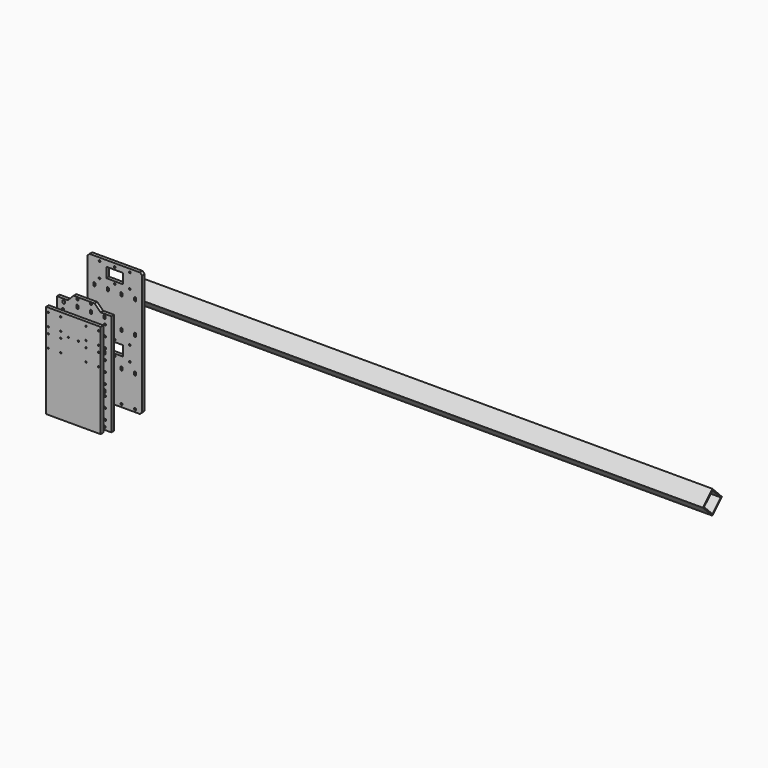
from build123d import *

# Parameters (mm, degrees)
F2_DEPTH  = 1380
F3_T      = -2.5
F4_R      = 2.25
F4_R_2    = 2.5
F4_R_3    = 2.5703929726
F4_R_4    = 2.4889347238
F5_DEPTH  = 8
F7_R      = 2.5
F7_R_2    = 2.05
F7_W      = 40
F7_H      = 24
F8_DEPTH  = 8
F10_W     = 130
F10_H     = 225
F10_R     = 1.65
F11_DEPTH = 8


# Not quite as in the source:
# - a feature names something its author has since deleted; it is built from what else it names


with BuildPart() as f2:
    # F1 (on Right) → F2 (new body)
    with BuildSketch(Plane.YZ):
        Polygon((165.6129737569, 100.5009111076), (137.3287025094, 128.785182355), (109.0444312619, 100.5009111076), (137.3287025094, 72.2166398601), align=None)
    extrude(amount=F2_DEPTH)

    # F3
    f3_openings = [f2.faces().sort_by_distance(p)[0] for p in [
        (0, 137.328703, 100.500911),
        (1380, 137.328703, 100.500911),
    ]]
    offset(amount=F3_T, openings=f3_openings)


with BuildPart() as f5:
    # F4 (on Front) → F5 (new body)
    with BuildSketch(Plane.XZ):
        Polygon((65, -121.7), (65, 121.7), (39, 121.7), (25, 135.7), (-25, 135.7), (-39, 121.7), (-65, 121.7), (-65, -121.7), (-45, -121.7), (-34, -131.8), (34, -131.8), (45, -121.7), align=None)
        with Locations((-50, -100.09)):
            Circle(F4_R, mode=Mode.SUBTRACT)
        with Locations((-48.5, -115.09)):
            Circle(F4_R_2, mode=Mode.SUBTRACT)
        with Locations((-50, -75.09)):
            Circle(F4_R, mode=Mode.SUBTRACT)
        with Locations((-16.18, -127.59)):
            Circle(F4_R_2, mode=Mode.SUBTRACT)
        with Locations((-16.18, -115.09)):
            Circle(F4_R_2, mode=Mode.SUBTRACT)
        with Locations((-50, -50.09)):
            Circle(F4_R, mode=Mode.SUBTRACT)
        with BuildLine():
            Line((-46, -38.512), (-46, -42.512))
            ThreePointArc((-46, -42.512), (-48.5, -45.012), (-51, -42.512))
            Line((-51, -42.512), (-51, -38.512))
            ThreePointArc((-51, -38.512), (-48.5, -36.012), (-46, -38.512))
        make_face(mode=Mode.SUBTRACT)
        with Locations((-50, -25.09)):
            Circle(F4_R, mode=Mode.SUBTRACT)
        with Locations((-50, -0.09)):
            Circle(F4_R, mode=Mode.SUBTRACT)
        with BuildLine():
            Line((-13.68, -38.512), (-13.68, -42.512))
            ThreePointArc((-13.68, -42.512), (-16.18, -45.012), (-18.68, -42.512))
            Line((-18.68, -42.512), (-18.68, -38.512))
            ThreePointArc((-18.68, -38.512), (-16.18, -36.012), (-13.68, -38.512))
        make_face(mode=Mode.SUBTRACT)
        with Locations((16.18, -127.59)):
            Circle(F4_R_2, mode=Mode.SUBTRACT)
        with Locations((16.18, -115.09)):
            Circle(F4_R_2, mode=Mode.SUBTRACT)
        with Locations((48.5, -115.09)):
            Circle(F4_R_2, mode=Mode.SUBTRACT)
        with Locations((50, -100.09)):
            Circle(F4_R, mode=Mode.SUBTRACT)
        with Locations((50, -75.09)):
            Circle(F4_R, mode=Mode.SUBTRACT)
        with BuildLine():
            Line((18.68, -38.512), (18.68, -42.512))
            ThreePointArc((18.68, -42.512), (16.18, -45.012), (13.68, -42.512))
            Line((13.68, -42.512), (13.68, -38.512))
            ThreePointArc((13.68, -38.512), (16.18, -36.012), (18.68, -38.512))
        make_face(mode=Mode.SUBTRACT)
        with BuildLine():
            Line((51, -38.512), (51, -42.512))
            ThreePointArc((51, -42.512), (48.5, -45.012), (46, -42.512))
            Line((46, -42.512), (46, -38.512))
            ThreePointArc((46, -38.512), (48.5, -36.012), (51, -38.512))
        make_face(mode=Mode.SUBTRACT)
        with Locations((50, -50.09)):
            Circle(F4_R, mode=Mode.SUBTRACT)
        with Locations((50, -25.09)):
            Circle(F4_R, mode=Mode.SUBTRACT)
        with Locations((50, -0.09)):
            Circle(F4_R, mode=Mode.SUBTRACT)
        with Locations((-50, 24.91)):
            Circle(F4_R, mode=Mode.SUBTRACT)
        with Locations((-50, 49.91)):
            Circle(F4_R, mode=Mode.SUBTRACT)
        with BuildLine():
            Line((-51, 38.512), (-51, 42.512))
            ThreePointArc((-51, 42.512), (-48.5, 45.012), (-46, 42.512))
            Line((-46, 42.512), (-46, 38.512))
            ThreePointArc((-46, 38.512), (-48.5, 36.012), (-51, 38.512))
        make_face(mode=Mode.SUBTRACT)
        with BuildLine():
            Line((-18.68, 38.512), (-18.68, 42.512))
            ThreePointArc((-18.68, 42.512), (-16.18, 45.012), (-13.68, 42.512))
            Line((-13.68, 42.512), (-13.68, 38.512))
            ThreePointArc((-13.68, 38.512), (-16.18, 36.012), (-18.68, 38.512))
        make_face(mode=Mode.SUBTRACT)
        with Locations((-50, 74.91)):
            Circle(F4_R, mode=Mode.SUBTRACT)
        with Locations((-50, 99.91)):
            Circle(F4_R, mode=Mode.SUBTRACT)
        with BuildLine():
            Line((-51, 113.09), (-51, 117.09))
            ThreePointArc((-51, 117.09), (-48.5, 119.59), (-46, 117.09))
            Line((-46, 117.09), (-46, 113.09))
            ThreePointArc((-46, 113.09), (-48.5, 110.59), (-51, 113.09))
        make_face(mode=Mode.SUBTRACT)
        with BuildLine():
            Line((-18.68, 113.09), (-18.68, 117.09))
            ThreePointArc((-18.68, 117.09), (-16.18, 119.59), (-13.68, 117.09))
            Line((-13.68, 117.09), (-13.68, 113.09))
            ThreePointArc((-13.68, 113.09), (-16.18, 110.59), (-18.68, 113.09))
        make_face(mode=Mode.SUBTRACT)
        with Locations((-16.18, 130.7444572449)):
            Circle(F4_R_3, mode=Mode.SUBTRACT)
        with BuildLine():
            Line((13.68, 38.512), (13.68, 42.512))
            ThreePointArc((13.68, 42.512), (16.18, 45.012), (18.68, 42.512))
            Line((18.68, 42.512), (18.68, 38.512))
            ThreePointArc((18.68, 38.512), (16.18, 36.012), (13.68, 38.512))
        make_face(mode=Mode.SUBTRACT)
        with Locations((50, 24.91)):
            Circle(F4_R, mode=Mode.SUBTRACT)
        with BuildLine():
            Line((46, 38.512), (46, 42.512))
            ThreePointArc((46, 42.512), (48.5, 45.012), (51, 42.512))
            Line((51, 42.512), (51, 38.512))
            ThreePointArc((51, 38.512), (48.5, 36.012), (46, 38.512))
        make_face(mode=Mode.SUBTRACT)
        with Locations((50, 49.91)):
            Circle(F4_R, mode=Mode.SUBTRACT)
        with BuildLine():
            Line((13.68, 113.09), (13.68, 117.09))
            ThreePointArc((13.68, 117.09), (16.18, 119.59), (18.68, 117.09))
            Line((18.68, 117.09), (18.68, 113.09))
            ThreePointArc((18.68, 113.09), (16.18, 110.59), (13.68, 113.09))
        make_face(mode=Mode.SUBTRACT)
        with Locations((16.18, 132.09)):
            Circle(F4_R_4, mode=Mode.SUBTRACT)
        with Locations((50, 74.91)):
            Circle(F4_R, mode=Mode.SUBTRACT)
        with Locations((50, 99.91)):
            Circle(F4_R, mode=Mode.SUBTRACT)
        with BuildLine():
            Line((46, 113.09), (46, 117.09))
            ThreePointArc((46, 117.09), (48.5, 119.59), (51, 117.09))
            Line((51, 117.09), (51, 113.09))
            ThreePointArc((51, 113.09), (48.5, 110.59), (46, 113.09))
        make_face(mode=Mode.SUBTRACT)
    extrude(amount=F5_DEPTH)


with BuildPart() as f8:
    # F7 (on offset) → F8 (new body)
    with BuildSketch(Plane.XZ.offset(-83)):
        Polygon((60, 175.09), (-60, 175.09), (-65, 170.09), (-65, -116.7), (-60, -121.7), (60, -121.7), (65, -116.7), (65, 170.09), align=None)
        with Locations((-48.51, -115.2)):
            Circle(F7_R, mode=Mode.SUBTRACT)
        with Locations((-16.17, -115.2)):
            Circle(F7_R, mode=Mode.SUBTRACT)
        with BuildLine():
            Line((-46.01, -38.73), (-46.01, -42.73))
            ThreePointArc((-46.01, -42.73), (-48.51, -45.23), (-51.01, -42.73))
            Line((-51.01, -42.73), (-51.01, -38.9570118877))
            ThreePointArc((-51.01, -38.9570118877), (-48.6287763125, -36.2274246067), (-46.01, -38.73))
        make_face(mode=Mode.SUBTRACT)
        with Locations((-36, -20)):
            Circle(F7_R_2, mode=Mode.SUBTRACT)
        with Locations((-36, 15)):
            Circle(F7_R_2, mode=Mode.SUBTRACT)
        with BuildLine():
            Line((-13.67, -38.73), (-13.67, -42.73))
            ThreePointArc((-13.67, -42.73), (-16.17, -45.23), (-18.67, -42.73))
            Line((-18.67, -42.73), (-18.67, -39.0080270306))
            ThreePointArc((-18.67, -39.0080270306), (-16.3169581646, -36.2261380315), (-13.67, -38.73))
        make_face(mode=Mode.SUBTRACT)
        with Locations((16.17, -115.2)):
            Circle(F7_R, mode=Mode.SUBTRACT)
        with Locations((48.51, -115.2)):
            Circle(F7_R, mode=Mode.SUBTRACT)
        with BuildLine():
            Line((18.67, -38.73), (18.67, -42.73))
            ThreePointArc((18.67, -42.73), (16.17, -45.23), (13.67, -42.73))
            Line((13.67, -42.73), (13.67, -39.0075720796))
            ThreePointArc((13.67, -39.0075720796), (13.6584102142, -38.8690010606), (13.6545429641, -38.73))
            ThreePointArc((13.6545429641, -38.73), (16.1545429641, -36.23), (18.6545429641, -38.73))
            Line((18.6545429641, -38.73), (18.67, -38.73))
        make_face(mode=Mode.SUBTRACT)
        with Locations((0, -20)):
            Circle(F7_R_2, mode=Mode.SUBTRACT)
        with Locations((0, -2.5)):
            Rectangle(F7_W, F7_H, mode=Mode.SUBTRACT)
        with Locations((0, 15)):
            Circle(F7_R_2, mode=Mode.SUBTRACT)
        with BuildLine():
            Line((51.01, -42.7297875421), (51.01, -42.73))
            ThreePointArc((51.01, -42.73), (48.1449929341, -45.2503029403), (46.01, -42.0877094524))
            Line((46.01, -42.0877094524), (46.01, -38.73))
            ThreePointArc((46.01, -38.73), (48.51, -36.23), (51.01, -38.73))
            Line((51.01, -38.73), (51.01, -42.7297875421))
        make_face(mode=Mode.SUBTRACT)
        with Locations((36, -20)):
            Circle(F7_R_2, mode=Mode.SUBTRACT)
        with Locations((36, 15)):
            Circle(F7_R_2, mode=Mode.SUBTRACT)
        with BuildLine():
            Line((-46.01, 42.0886284048), (-46.01, 38.512))
            ThreePointArc((-46.01, 38.512), (-48.51, 36.012), (-51.01, 38.512))
            ThreePointArc((-51.01, 38.512), (-51.0009654295, 38.7243469541), (-50.9739270169, 38.9351591373))
            Line((-50.9739270169, 38.9351591373), (-50.9739270169, 42.5117875421))
            ThreePointArc((-50.9739270169, 42.5117875421), (-48.4739270169, 45.0117875421), (-45.9739270169, 42.5117875421))
            ThreePointArc((-45.9739270169, 42.5117875421), (-45.9829615873, 42.299440588), (-46.01, 42.0886284048))
        make_face(mode=Mode.SUBTRACT)
        with BuildLine():
            Line((-13.67, 42.1039142989), (-13.67, 38.512))
            ThreePointArc((-13.67, 38.512), (-16.17, 36.012), (-18.67, 38.512))
            ThreePointArc((-18.67, 38.512), (-18.6616117976, 38.7166231899), (-18.6365034801, 38.9198732432))
            Line((-18.6365034801, 38.9198732432), (-18.6365034801, 42.5117875421))
            ThreePointArc((-18.6365034801, 42.5117875421), (-16.1365034801, 45.0117875421), (-13.6365034801, 42.5117875421))
            ThreePointArc((-13.6365034801, 42.5117875421), (-13.6448916825, 42.3071643522), (-13.67, 42.1039142989))
        make_face(mode=Mode.SUBTRACT)
        with BuildLine():
            Line((-51.01, 113.09), (-51.01, 116.9834371618))
            ThreePointArc((-51.01, 116.9834371618), (-48.5632935076, 119.5917025084), (-46.007729903, 117.09))
            Line((-46.007729903, 117.09), (-46.007729903, 113.09))
            ThreePointArc((-46.007729903, 113.09), (-48.507729903, 110.59), (-51.007729903, 113.09))
            Line((-51.007729903, 113.09), (-51.01, 113.09))
        make_face(mode=Mode.SUBTRACT)
        with Locations((-36, 131.59)):
            Circle(F7_R_2, mode=Mode.SUBTRACT)
        with Locations((-36, 167.59)):
            Circle(F7_R_2, mode=Mode.SUBTRACT)
        with BuildLine():
            ThreePointArc((-13.667729903, 113.09), (-16.167729903, 110.59), (-18.667729903, 113.09))
            Line((-18.667729903, 113.09), (-18.67, 113.09))
            Line((-18.67, 113.09), (-18.67, 116.9834371618))
            ThreePointArc((-18.67, 116.9834371618), (-16.2232935076, 119.5917025084), (-13.667729903, 117.09))
            Line((-13.667729903, 117.09), (-13.667729903, 113.09))
        make_face(mode=Mode.SUBTRACT)
        with BuildLine():
            Line((18.67, 42.1537611834), (18.67, 38.512))
            ThreePointArc((18.67, 38.512), (16.17, 36.012), (13.67, 38.512))
            ThreePointArc((13.67, 38.512), (13.676450669, 38.6914762762), (13.695769387, 38.8700263587))
            Line((13.695769387, 38.8700263587), (13.695769387, 42.5117875421))
            ThreePointArc((13.695769387, 42.5117875421), (16.195769387, 45.0117875421), (18.695769387, 42.5117875421))
            ThreePointArc((18.695769387, 42.5117875421), (18.689318718, 42.3323112659), (18.67, 42.1537611834))
        make_face(mode=Mode.SUBTRACT)
        with BuildLine():
            Line((51.01, 42.0596454226), (51.01, 38.512))
            ThreePointArc((51.01, 38.512), (48.51, 36.012), (46.01, 38.512))
            ThreePointArc((46.01, 38.512), (46.020327939, 38.7390088733), (46.0512264229, 38.9641421196))
            Line((46.0512264229, 38.9641421196), (46.0512264229, 42.5117875421))
            ThreePointArc((46.0512264229, 42.5117875421), (48.5512264228, 45.0117875421), (51.0512264228, 42.5117875421))
            ThreePointArc((51.0512264228, 42.5117875421), (51.0408984839, 42.2847786688), (51.01, 42.0596454226))
        make_face(mode=Mode.SUBTRACT)
        with BuildLine():
            ThreePointArc((18.68, 113.09), (16.18, 110.59), (13.68, 113.09))
            Line((13.68, 113.09), (13.67, 113.09))
            Line((13.67, 113.09), (13.67, 116.8124279204))
            ThreePointArc((13.67, 116.8124279204), (13.6584102142, 116.9509989394), (13.6545429641, 117.09))
            ThreePointArc((13.6545429641, 117.09), (16.1545429641, 119.59), (18.6545429641, 117.09))
            Line((18.6545429641, 117.09), (18.67, 117.09))
            Line((18.67, 117.09), (18.68, 117.09))
            Line((18.68, 117.09), (18.68, 113.09))
        make_face(mode=Mode.SUBTRACT)
        with Locations((0, 131.59)):
            Circle(F7_R_2, mode=Mode.SUBTRACT)
        with Locations((0, 149.09)):
            Rectangle(F7_W, F7_H, mode=Mode.SUBTRACT)
        with Locations((0, 166.59)):
            Circle(F7_R_2, mode=Mode.SUBTRACT)
        with BuildLine():
            Line((51.01, 117.09), (51.01, 113.09))
            ThreePointArc((51.01, 113.09), (48.51, 110.59), (46.01, 113.09))
            Line((46.01, 113.09), (46.01, 117.09))
            ThreePointArc((46.01, 117.09), (48.51, 119.59), (51.01, 117.09))
        make_face(mode=Mode.SUBTRACT)
        with Locations((36, 132.59)):
            Circle(F7_R_2, mode=Mode.SUBTRACT)
        with Locations((36, 167.59)):
            Circle(F7_R_2, mode=Mode.SUBTRACT)
    extrude(amount=-F8_DEPTH)


with BuildPart() as f11:
    # F10 (on offset) → F11 (new body)
    with BuildSketch(Plane.XZ.offset(32)):
        Rectangle(F10_W, F10_H)
        with Locations((-60, 27.5)):
            Circle(F10_R, mode=Mode.SUBTRACT)
        with Locations((-30, 27.5)):
            Circle(F10_R, mode=Mode.SUBTRACT)
        with Locations((-60, 57.5)):
            Circle(F10_R, mode=Mode.SUBTRACT)
        with Locations((-60, 72.5)):
            Circle(F10_R, mode=Mode.SUBTRACT)
        with Locations((-60, 102.5)):
            Circle(F10_R, mode=Mode.SUBTRACT)
        with Locations((-30, 57.5)):
            Circle(F10_R, mode=Mode.SUBTRACT)
        with Locations((-30, 72.5)):
            Circle(F10_R, mode=Mode.SUBTRACT)
        with Locations((-12, 65.5)):
            Circle(F10_R, mode=Mode.SUBTRACT)
        with Locations((-30, 102.5)):
            Circle(F10_R, mode=Mode.SUBTRACT)
        with Locations((30, 27.5)):
            Circle(F10_R, mode=Mode.SUBTRACT)
        with Locations((60, 27.5)):
            Circle(F10_R, mode=Mode.SUBTRACT)
        with Locations((12, 65.5)):
            Circle(F10_R, mode=Mode.SUBTRACT)
        with Locations((30, 57.5)):
            Circle(F10_R, mode=Mode.SUBTRACT)
        with Locations((30, 72.5)):
            Circle(F10_R, mode=Mode.SUBTRACT)
        with Locations((30, 102.5)):
            Circle(F10_R, mode=Mode.SUBTRACT)
        with Locations((60, 57.5)):
            Circle(F10_R, mode=Mode.SUBTRACT)
        with Locations((60, 72.5)):
            Circle(F10_R, mode=Mode.SUBTRACT)
        with Locations((60, 102.5)):
            Circle(F10_R, mode=Mode.SUBTRACT)
    extrude(amount=F11_DEPTH)


solid = Compound([f2.part, f5.part, f8.part, f11.part])
